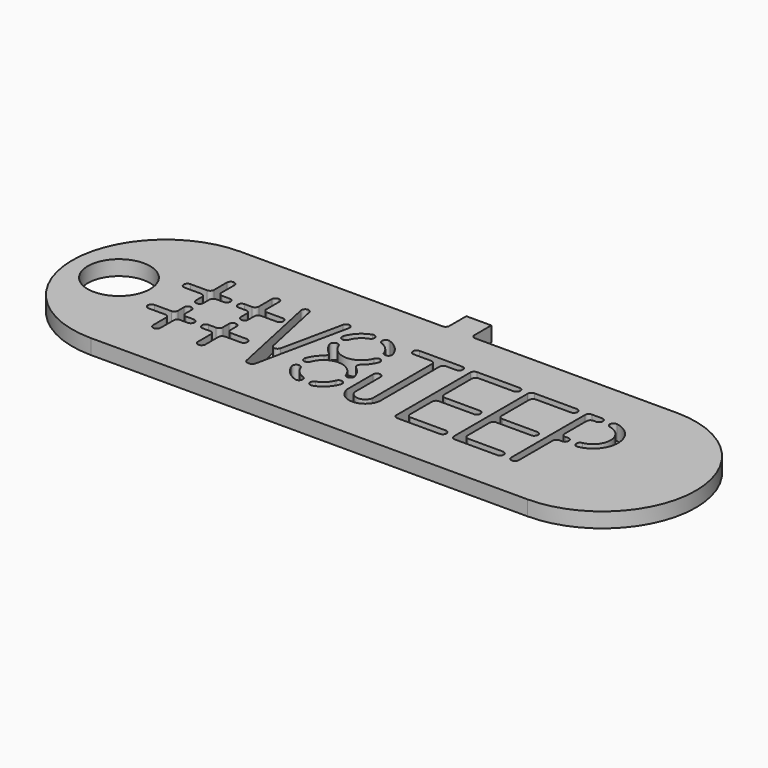
from build123d import *

# Parameters (mm, degrees)
F0_R        = 3.175
F1_DEPTH    = 1.524
F2_T1_DEPTH = 1.524
F2_T3_DEPTH = 10.4029181171
F2_T5_DEPTH = 3.429
F2_T7_DEPTH = 4.4158412882
F3_R        = 0.38
F4_R        = 0.38


# Not quite as in the source:
# - a fillet or chamfer that OpenCascade refuses, or shapes differently, is made with other operations: its cross-section is extruded or revolved along the edge and cut away or added
# - a fillet or chamfer is up to 0.001 mm smaller than in the source, because OpenCascade refuses the exact size


with BuildPart() as f1:
    # F0 (on Top) → F1 (new body)
    with BuildSketch(Plane.XY):
        with BuildLine():
            Line((30.48, 19.05), (9.525, 19.05))
            ThreePointArc((9.525, 19.05), (0, 9.525), (9.525, 0))
            Line((9.525, 0), (53.975, 0))
            ThreePointArc((53.975, 0), (63.5, 9.525), (53.975, 19.05))
            Line((53.975, 19.05), (33.02, 19.05))
            Line((33.02, 19.05), (33.02, 21.59))
            Line((33.02, 21.59), (30.48, 21.59))
            Line((30.48, 21.59), (30.48, 19.05))
        make_face()
        Polygon((9.525, 7.6261373708), (11.990133673, 7.6261373708), (11.990133673, 9.1501373708), (12.752133673, 9.1501373708), (12.752133673, 7.6261373708), (14.276133673, 7.6261373708), (14.276133673, 6.8641373708), (12.752133673, 6.8641373708), (12.752133673, 4.445), (11.990133673, 4.445), (11.990133673, 6.8641373708), (9.525, 6.8641373708), align=None, mode=Mode.SUBTRACT)
        with Locations((4.7625, 9.525)):
            Circle(F0_R, mode=Mode.SUBTRACT)
        Polygon((16.562133673, 6.8641373708), (15.038133673, 6.8641373708), (15.038133673, 7.6261373708), (16.562133673, 7.6261373708), (16.562133673, 9.1501373708), (17.324133673, 9.1501373708), (17.324133673, 7.6261373708), (19.685, 7.6261373708), (19.685, 6.8641373708), (17.324133673, 6.8641373708), (17.324133673, 4.445), (16.562133673, 4.445), align=None, mode=Mode.SUBTRACT)
        with BuildLine():
            ThreePointArc((25.6528369587, 6.6981185685), (26.1772344094, 5.7531270917), (27.1313334392, 5.245488816))
            Line((27.1313334392, 5.245488816), (27.1313334392, 4.4723545693))
            ThreePointArc((27.1313334392, 4.4723545693), (25.6382729221, 5.2144262391), (24.8776434838, 6.6981185685))
            Line((24.8776434838, 6.6981185685), (25.6528369587, 6.6981185685))
        make_face(mode=Mode.SUBTRACT)
        with BuildLine():
            Line((27.8933334392, 4.4723545693), (27.8933334392, 5.245488816))
            ThreePointArc((27.8933334392, 5.245488816), (28.8528284175, 5.7584497745), (29.3750644231, 6.7129282251))
            Line((29.3750644231, 6.7129282251), (30.1493072196, 6.7129282251))
            ThreePointArc((30.1493072196, 6.7129282251), (29.3917173839, 5.2196984943), (27.8933334392, 4.4723545693))
        make_face(mode=Mode.SUBTRACT)
        Polygon((21.6525053587, 4.445), (19.4935053587, 14.605), (20.2555053587, 14.605), (22.0335053587, 6.3180097573), (23.8115053587, 14.605), (24.5735053587, 14.605), (22.4145053587, 4.445), align=None, mode=Mode.SUBTRACT)
        with BuildLine():
            ThreePointArc((26.3764109066, 9.525), (25.3757333504, 10.3418079499), (24.876256228, 11.5330482291))
            Line((24.876256228, 11.5330482291), (25.6508718996, 11.5330482291))
            ThreePointArc((25.6508718996, 11.5330482291), (27.5215165568, 10.0330221339), (29.3776125895, 11.5510133188))
            Line((29.3776125895, 11.5510133188), (30.1511078343, 11.5510133188))
            ThreePointArc((30.1511078343, 11.5510133188), (29.6543574157, 10.3490939978), (28.6482559717, 9.525))
            ThreePointArc((28.6482559717, 9.525), (29.6615736807, 8.6911312118), (30.1545242164, 7.4749282251))
            Line((30.1545242164, 7.4749282251), (29.3824425545, 7.4749282251))
            ThreePointArc((29.3824425545, 7.4749282251), (27.5047961864, 9.0169850891), (25.6394110002, 7.4601185685))
            Line((25.6394110002, 7.4601185685), (24.8681506803, 7.4601185685))
            ThreePointArc((24.8681506803, 7.4601185685), (25.3586777482, 8.6851039905), (26.3764109066, 9.525))
        make_face(mode=Mode.SUBTRACT)
        with BuildLine():
            Line((30.9413334392, 5.8339602692), (30.9413334392, 9.525))
            Line((30.9413334392, 9.525), (31.7033334392, 9.525))
            Line((31.7033334392, 9.525), (31.7033334392, 5.8339602692))
            ThreePointArc((31.7033334392, 5.8339602692), (32.5923334392, 5.1729728532), (33.4813334392, 5.8339602692))
            Line((33.4813334392, 5.8339602692), (33.4813334392, 13.843))
            Line((33.4813334392, 13.843), (30.9413334392, 13.843))
            Line((30.9413334392, 13.843), (30.9413334392, 14.605))
            Line((30.9413334392, 14.605), (36.0213334392, 14.605))
            Line((36.0213334392, 14.605), (36.0213334392, 13.843))
            Line((36.0213334392, 13.843), (34.2433334392, 13.843))
            Line((34.2433334392, 13.843), (34.2433334392, 5.8339602692))
            ThreePointArc((34.2433334392, 5.8339602692), (32.5923334392, 4.4338967074), (30.9413334392, 5.8339602692))
        make_face(mode=Mode.SUBTRACT)
        Polygon((41.8633334392, 14.605), (41.8633334392, 13.843), (37.5453334392, 13.843), (37.5453334392, 9.5561961154), (41.8633334392, 9.5561961154), (41.8633334392, 8.7941961154), (37.5453334392, 8.7941961154), (37.5453334392, 5.207), (41.8633334392, 5.207), (41.8633334392, 4.445), (36.7833334392, 4.445), (36.7833334392, 14.605), align=None, mode=Mode.SUBTRACT)
        Polygon((42.6253334392, 4.445), (42.6253334392, 14.605), (47.7053334392, 14.605), (47.7053334392, 13.843), (43.3873334392, 13.843), (43.3873334392, 9.5561961154), (47.7053334392, 9.5561961154), (47.7053334392, 8.7941961154), (43.3873334392, 8.7941961154), (43.3873334392, 5.207), (47.7053334392, 5.207), (47.7053334392, 4.445), align=None, mode=Mode.SUBTRACT)
        Polygon((49.2293334392, 4.445), (48.4673334392, 4.445), (48.4673334392, 14.605), (50.2805225551, 14.605), (50.2805225551, 13.8435801491), (49.2293334392, 13.843), (49.2293334392, 10.287), (50.2624474466, 10.287), (50.2624474466, 9.525), (49.2293334392, 9.525), align=None, mode=Mode.SUBTRACT)
        Polygon((11.990133673, 12.1981373708), (11.990133673, 14.605), (12.752133673, 14.605), (12.752133673, 12.1981373708), (14.276133673, 12.1981373708), (14.276133673, 11.4361373708), (12.752133673, 11.4361373708), (12.752133673, 9.9121373708), (11.990133673, 9.9121373708), (11.990133673, 11.4361373708), (9.525, 11.4361373708), (9.525, 12.1981373708), align=None, mode=Mode.SUBTRACT)
        Polygon((16.562133673, 12.1981373708), (16.562133673, 14.605), (17.324133673, 14.605), (17.324133673, 12.1981373708), (19.685, 12.1981373708), (19.685, 11.4361373708), (17.324133673, 11.4361373708), (17.324133673, 9.9121373708), (16.562133673, 9.9121373708), (16.562133673, 11.4361373708), (15.038133673, 11.4361373708), (15.038133673, 12.1981373708), align=None, mode=Mode.SUBTRACT)
        with BuildLine():
            ThreePointArc((24.8693416567, 12.2950482291), (25.6185493529, 13.8158899953), (27.1330227926, 14.5778887161))
            Line((27.1330227926, 14.5778887161), (27.1330227926, 13.8048552256))
            ThreePointArc((27.1330227926, 13.8048552256), (26.1572966965, 13.2769923174), (25.6410927913, 12.2950482291))
            Line((25.6410927913, 12.2950482291), (24.8693416567, 12.2950482291))
        make_face(mode=Mode.SUBTRACT)
        with BuildLine():
            ThreePointArc((29.3800566549, 12.3130133188), (28.8621381004, 13.2822664827), (27.8950224806, 13.8041656137))
            Line((27.8950224806, 13.8041656137), (27.8950227926, 14.5774010417))
            ThreePointArc((27.8950227926, 14.5774010417), (29.4009269225, 13.8211101016), (30.1528360449, 12.3130133188))
            Line((30.1528360449, 12.3130133188), (29.3800566549, 12.3130133188))
        make_face(mode=Mode.SUBTRACT)
        with BuildLine():
            ThreePointArc((51.0073334392, 14.605), (53.5473334392, 12.065), (51.0073334392, 9.525))
            Line((51.0073334392, 9.525), (51.0073334392, 10.287))
            ThreePointArc((51.0073334392, 10.287), (52.7853334392, 12.065), (51.0073334392, 13.843))
            Line((51.0073334392, 13.843), (51.0073334392, 14.605))
        make_face(mode=Mode.SUBTRACT)
    extrude(amount=F1_DEPTH)

    # F2: fillet of radius 0.381 on 77 edges, made by hand

    # F2_s2 → F2_t1 (join)
    with BuildSketch(Plane.XY):
        with BuildLine():
            ThreePointArc((24.103035572, 14.605), (24.3991216953, 14.4637790808), (24.4757140942, 14.144805814))
            Line((24.4757140942, 14.144805814), (24.5735053587, 14.605))
            Line((24.5735053587, 14.605), (24.103035572, 14.605))
        make_face()
        with BuildLine():
            ThreePointArc((20.3201017736, 14.3039258381), (20.1870677408, 14.5203214001), (19.9475794784, 14.605))
            Line((19.9475794784, 14.605), (20.2555053587, 14.605))
            Line((20.2555053587, 14.605), (20.3201017736, 14.3039258381))
        make_face()
        with BuildLine():
            ThreePointArc((23.7469089438, 14.3039258381), (23.8799429766, 14.5203214001), (24.119431239, 14.605))
            Line((24.119431239, 14.605), (23.8115053587, 14.605))
            Line((23.8115053587, 14.605), (23.7469089438, 14.3039258381))
        make_face()
        with BuildLine():
            ThreePointArc((19.5912966232, 14.144805814), (19.6678890221, 14.4637790808), (19.9639751454, 14.605))
            Line((19.9639751454, 14.605), (19.4935053587, 14.605))
            Line((19.4935053587, 14.605), (19.5912966232, 14.144805814))
        make_face()
        with BuildLine():
            ThreePointArc((21.9610501454, 4.445), (21.7212710646, 4.5299138767), (21.5883716232, 4.746805814))
            Line((21.5883716232, 4.746805814), (21.6525053587, 4.445))
            Line((21.6525053587, 4.445), (21.9610501454, 4.445))
        make_face()
        with BuildLine():
            ThreePointArc((22.4786390942, 4.746805814), (22.3457396527, 4.5299138767), (22.105960572, 4.445))
            Line((22.105960572, 4.445), (22.4145053587, 4.445))
            Line((22.4145053587, 4.445), (22.4786390942, 4.746805814))
        make_face()
        with BuildLine():
            ThreePointArc((35.6403334392, 14.605), (35.9097411228, 14.4934076836), (36.0213334392, 14.224))
            Line((36.0213334392, 14.224), (36.0213334392, 14.605))
            Line((36.0213334392, 14.605), (35.6403334392, 14.605))
        make_face()
        with BuildLine():
            ThreePointArc((36.0213334392, 14.224), (35.9097411228, 13.9545923164), (35.6403334392, 13.843))
            Line((35.6403334392, 13.843), (36.0213334392, 13.843))
            Line((36.0213334392, 13.843), (36.0213334392, 14.224))
        make_face()
        with BuildLine():
            ThreePointArc((31.3223334392, 13.843), (31.0529257555, 13.9545923164), (30.9413334392, 14.224))
            Line((30.9413334392, 14.224), (30.9413334392, 13.843))
            Line((30.9413334392, 13.843), (31.3223334392, 13.843))
        make_face()
        with BuildLine():
            ThreePointArc((30.9413334392, 14.224), (31.0529257555, 14.4934076836), (31.3223334392, 14.605))
            Line((31.3223334392, 14.605), (30.9413334392, 14.605))
            Line((30.9413334392, 14.605), (30.9413334392, 14.224))
        make_face()
        with BuildLine():
            ThreePointArc((30.9413334392, 9.144), (31.0529257555, 9.4134076836), (31.3223334392, 9.525))
            Line((31.3223334392, 9.525), (30.9413334392, 9.525))
            Line((30.9413334392, 9.525), (30.9413334392, 9.144))
        make_face()
        with BuildLine():
            ThreePointArc((31.3223334392, 9.525), (31.5917411228, 9.4134076836), (31.7033334392, 9.144))
            Line((31.7033334392, 9.144), (31.7033334392, 9.525))
            Line((31.7033334392, 9.525), (31.3223334392, 9.525))
        make_face()
        with BuildLine():
            ThreePointArc((41.4823334392, 14.605), (41.7517411228, 14.4934076836), (41.8633334392, 14.224))
            Line((41.8633334392, 14.224), (41.8633334392, 14.605))
            Line((41.8633334392, 14.605), (41.4823334392, 14.605))
        make_face()
        with BuildLine():
            ThreePointArc((41.4823334392, 9.5561961154), (41.7517411228, 9.444603799), (41.8633334392, 9.1751961154))
            Line((41.8633334392, 9.1751961154), (41.8633334392, 9.5561961154))
            Line((41.8633334392, 9.5561961154), (41.4823334392, 9.5561961154))
        make_face()
        with BuildLine():
            ThreePointArc((41.4823334392, 5.207), (41.7517411228, 5.0954076836), (41.8633334392, 4.826))
            Line((41.8633334392, 4.826), (41.8633334392, 5.207))
            Line((41.8633334392, 5.207), (41.4823334392, 5.207))
        make_face()
        with BuildLine():
            ThreePointArc((37.1643334392, 14.605), (36.8949257555, 14.4934076836), (36.7833334392, 14.224))
            Line((36.7833334392, 14.224), (36.7833334392, 14.605))
            Line((36.7833334392, 14.605), (37.1643334392, 14.605))
        make_face()
        with BuildLine():
            ThreePointArc((37.1643334392, 4.445), (36.8949257555, 4.5565923164), (36.7833334392, 4.826))
            Line((36.7833334392, 4.826), (36.7833334392, 4.445))
            Line((36.7833334392, 4.445), (37.1643334392, 4.445))
        make_face()
        with BuildLine():
            ThreePointArc((42.6253334392, 4.826), (42.7369257555, 4.5565923164), (43.0063334392, 4.445))
            Line((43.0063334392, 4.445), (42.6253334392, 4.445))
            Line((42.6253334392, 4.445), (42.6253334392, 4.826))
        make_face()
        with BuildLine():
            ThreePointArc((41.8633334392, 4.826), (41.7517411228, 4.5565923164), (41.4823334392, 4.445))
            Line((41.4823334392, 4.445), (41.8633334392, 4.445))
            Line((41.8633334392, 4.445), (41.8633334392, 4.826))
        make_face()
        with BuildLine():
            ThreePointArc((41.8633334392, 9.1751961154), (41.7517411228, 8.9057884318), (41.4823334392, 8.7941961154))
            Line((41.4823334392, 8.7941961154), (41.8633334392, 8.7941961154))
            Line((41.8633334392, 8.7941961154), (41.8633334392, 9.1751961154))
        make_face()
        with BuildLine():
            ThreePointArc((41.8633334392, 14.224), (41.7517411228, 13.9545923164), (41.4823334392, 13.843))
            Line((41.4823334392, 13.843), (41.8633334392, 13.843))
            Line((41.8633334392, 13.843), (41.8633334392, 14.224))
        make_face()
        with BuildLine():
            ThreePointArc((47.7053334392, 4.826), (47.5937411228, 4.5565923164), (47.3243334392, 4.445))
            Line((47.3243334392, 4.445), (47.7053334392, 4.445))
            Line((47.7053334392, 4.445), (47.7053334392, 4.826))
        make_face()
        with BuildLine():
            ThreePointArc((47.7053334392, 9.1751961154), (47.5937411228, 8.9057884318), (47.3243334392, 8.7941961154))
            Line((47.3243334392, 8.7941961154), (47.7053334392, 8.7941961154))
            Line((47.7053334392, 8.7941961154), (47.7053334392, 9.1751961154))
        make_face()
        with BuildLine():
            ThreePointArc((47.7053334392, 14.224), (47.5937411228, 13.9545923164), (47.3243334392, 13.843))
            Line((47.3243334392, 13.843), (47.7053334392, 13.843))
            Line((47.7053334392, 13.843), (47.7053334392, 14.224))
        make_face()
        with BuildLine():
            ThreePointArc((42.6253334392, 14.224), (42.7369257555, 14.4934076836), (43.0063334392, 14.605))
            Line((43.0063334392, 14.605), (42.6253334392, 14.605))
            Line((42.6253334392, 14.605), (42.6253334392, 14.224))
        make_face()
        with BuildLine():
            ThreePointArc((47.3243334392, 5.207), (47.5937411228, 5.0954076836), (47.7053334392, 4.826))
            Line((47.7053334392, 4.826), (47.7053334392, 5.207))
            Line((47.7053334392, 5.207), (47.3243334392, 5.207))
        make_face()
        with BuildLine():
            ThreePointArc((47.3243334392, 9.5561961154), (47.5937411228, 9.444603799), (47.7053334392, 9.1751961154))
            Line((47.7053334392, 9.1751961154), (47.7053334392, 9.5561961154))
            Line((47.7053334392, 9.5561961154), (47.3243334392, 9.5561961154))
        make_face()
        with BuildLine():
            ThreePointArc((47.3243334392, 14.605), (47.5937411228, 14.4934076836), (47.7053334392, 14.224))
            Line((47.7053334392, 14.224), (47.7053334392, 14.605))
            Line((47.7053334392, 14.605), (47.3243334392, 14.605))
        make_face()
        with BuildLine():
            ThreePointArc((49.8995225551, 14.605), (50.1689302387, 14.4934076836), (50.2805225551, 14.224))
            Line((50.2805225551, 14.224), (50.2805225551, 14.605))
            Line((50.2805225551, 14.605), (49.8995225551, 14.605))
        make_face()
        with BuildLine():
            ThreePointArc((49.8814474466, 10.287), (50.1508551302, 10.1754076836), (50.2624474466, 9.906))
            Line((50.2624474466, 9.906), (50.2624474466, 10.287))
            Line((50.2624474466, 10.287), (49.8814474466, 10.287))
        make_face()
        with BuildLine():
            ThreePointArc((50.2624474466, 9.906), (50.1508551302, 9.6365923164), (49.8814474466, 9.525))
            Line((49.8814474466, 9.525), (50.2624474466, 9.525))
            Line((50.2624474466, 9.525), (50.2624474466, 9.906))
        make_face()
        with BuildLine():
            ThreePointArc((48.8483334392, 4.445), (49.1177411228, 4.5565923164), (49.2293334392, 4.826))
            Line((49.2293334392, 4.826), (49.2293334392, 4.445))
            Line((49.2293334392, 4.445), (48.8483334392, 4.445))
        make_face()
        with BuildLine():
            ThreePointArc((51.4555687333, 9.5648629795), (51.14384995, 9.6476698719), (51.0073334392, 9.9398835326))
            Line((51.0073334392, 9.9398835326), (51.0073334392, 9.525))
            ThreePointArc((51.0073334392, 9.525), (51.2323356258, 9.5349853724), (51.4555687333, 9.5648629795))
        make_face()
        with BuildLine():
            ThreePointArc((51.321098145, 13.8150959143), (51.0961197784, 13.9456329782), (51.0073334392, 14.1901164674))
            Line((51.0073334392, 14.1901164674), (51.0073334392, 13.843))
            ThreePointArc((51.0073334392, 13.843), (51.1648349698, 13.8360102393), (51.321098145, 13.8150959143))
        make_face()
        with BuildLine():
            ThreePointArc((51.321098145, 10.3149040857), (51.0961197784, 10.1843670218), (51.0073334392, 9.9398835326))
            Line((51.0073334392, 9.9398835326), (51.0073334392, 10.287))
            ThreePointArc((51.0073334392, 10.287), (51.1648349698, 10.2939897607), (51.321098145, 10.3149040857))
        make_face()
        with BuildLine():
            ThreePointArc((51.0073334392, 14.1901164674), (51.14384995, 14.4823301281), (51.4555687333, 14.5651370205))
            ThreePointArc((51.4555687333, 14.5651370205), (51.2323356258, 14.5950146276), (51.0073334392, 14.605))
            Line((51.0073334392, 14.605), (51.0073334392, 14.1901164674))
        make_face()
        with BuildLine():
            ThreePointArc((48.4673334392, 14.224), (48.5789257555, 14.4934076836), (48.8483334392, 14.605))
            Line((48.8483334392, 14.605), (48.4673334392, 14.605))
            Line((48.4673334392, 14.605), (48.4673334392, 14.224))
        make_face()
        with BuildLine():
            ThreePointArc((48.8483334392, 4.445), (48.5789257555, 4.5565923164), (48.4673334392, 4.826))
            Line((48.4673334392, 4.826), (48.4673334392, 4.445))
            Line((48.4673334392, 4.445), (48.8483334392, 4.445))
        make_face()
        with BuildLine():
            ThreePointArc((29.6738992595, 7.4749282251), (29.4526284326, 7.5457666202), (29.3136382895, 7.7319401876))
            ThreePointArc((29.3136382895, 7.7319401876), (29.3525328615, 7.6046368702), (29.3824425545, 7.4749282251))
            Line((29.3824425545, 7.4749282251), (29.6738992595, 7.4749282251))
        make_face()
        with BuildLine():
            ThreePointArc((30.0341602296, 7.9799162626), (29.9840608644, 7.6346573982), (29.6738992595, 7.4749282251))
            Line((29.6738992595, 7.4749282251), (30.1545242164, 7.4749282251))
            ThreePointArc((30.1545242164, 7.4749282251), (30.1066585131, 7.7303578338), (30.0341602296, 7.9799162626))
        make_face()
        with BuildLine():
            ThreePointArc((29.6611200796, 6.7129282251), (29.9731261354, 6.5505905702), (30.0192511863, 6.2019162626))
            ThreePointArc((30.0192511863, 6.2019162626), (30.0969394668, 6.4542001203), (30.1493072196, 6.7129282251))
            Line((30.1493072196, 6.7129282251), (29.6611200796, 6.7129282251))
        make_face()
        with BuildLine():
            ThreePointArc((27.8933334392, 4.9567385309), (28.0543629866, 4.6456533336), (28.4013334392, 4.5975282861))
            ThreePointArc((28.4013334392, 4.5975282861), (28.150410327, 4.5224543091), (27.8933334392, 4.4723545693))
            Line((27.8933334392, 4.4723545693), (27.8933334392, 4.9567385309))
        make_face()
        with BuildLine():
            ThreePointArc((27.8933334392, 4.9567385309), (27.9632482418, 5.1767089835), (28.1473334392, 5.3159487758))
            ThreePointArc((28.1473334392, 5.3159487758), (28.0215535796, 5.2763203306), (27.8933334392, 5.245488816))
            Line((27.8933334392, 5.245488816), (27.8933334392, 4.9567385309))
        make_face()
        with BuildLine():
            ThreePointArc((29.3029889728, 6.4619401876), (29.4424577345, 6.6439342809), (29.6611200796, 6.7129282251))
            Line((29.6611200796, 6.7129282251), (29.3750644231, 6.7129282251))
            ThreePointArc((29.3750644231, 6.7129282251), (29.3433323497, 6.5861977658), (29.3029889728, 6.4619401876))
        make_face()
        with BuildLine():
            ThreePointArc((25.3689810393, 6.6981185685), (25.5865655391, 6.6298772382), (25.7262064393, 6.4495988071))
            ThreePointArc((25.7262064393, 6.4495988071), (25.6852912508, 6.5726097498), (25.6528369587, 6.6981185685))
            Line((25.6528369587, 6.6981185685), (25.3689810393, 6.6981185685))
        make_face()
        with BuildLine():
            ThreePointArc((27.1313334392, 4.9567385309), (27.0614186365, 5.1767089835), (26.8773334392, 5.3159487758))
            ThreePointArc((26.8773334392, 5.3159487758), (27.0031132987, 5.2763203306), (27.1313334392, 5.245488816))
            Line((27.1313334392, 5.245488816), (27.1313334392, 4.9567385309))
        make_face()
        with BuildLine():
            ThreePointArc((27.1313334392, 4.9567385309), (26.9703038917, 4.6456533336), (26.6233334392, 4.5975282861))
            ThreePointArc((26.6233334392, 4.5975282861), (26.8742565513, 4.5224543091), (27.1313334392, 4.4723545693))
            Line((27.1313334392, 4.4723545693), (27.1313334392, 4.9567385309))
        make_face()
        with BuildLine():
            ThreePointArc((25.0117556393, 6.1846383299), (25.0562223697, 6.5347030683), (25.3689810393, 6.6981185685))
            Line((25.3689810393, 6.6981185685), (24.8776434838, 6.6981185685))
            ThreePointArc((24.8776434838, 6.6981185685), (24.9318956433, 6.4380342873), (25.0117556393, 6.1846383299))
        make_face()
        with BuildLine():
            ThreePointArc((25.3457273114, 7.4601185685), (25.5680581132, 7.5317158947), (25.7068283327, 7.7195988071))
            ThreePointArc((25.7068283327, 7.7195988071), (25.6685493411, 7.5910461353), (25.6394110002, 7.4601185685))
            Line((25.6394110002, 7.4601185685), (25.3457273114, 7.4601185685))
        make_face()
        with BuildLine():
            ThreePointArc((25.3457273114, 7.4601185685), (25.0363246376, 7.6187877667), (24.9846262901, 7.9626383299))
            ThreePointArc((24.9846262901, 7.9626383299), (24.9142104951, 7.7142011021), (24.8681506803, 7.4601185685))
            Line((24.8681506803, 7.4601185685), (25.3457273114, 7.4601185685))
        make_face()
        with BuildLine():
            ThreePointArc((25.0079167025, 11.0210562673), (25.0533854328, 11.3702832659), (25.365690522, 11.5330482291))
            Line((25.365690522, 11.5330482291), (24.876256228, 11.5330482291))
            ThreePointArc((24.876256228, 11.5330482291), (24.9293693571, 11.2737820006), (25.0079167025, 11.0210562673))
        make_face()
        with BuildLine():
            ThreePointArc((25.365690522, 11.5330482291), (25.5839255588, 11.4643533183), (25.7234643415, 11.2830401909))
            ThreePointArc((25.7234643415, 11.2830401909), (25.6828924193, 11.4068027155), (25.6508718996, 11.5330482291))
            Line((25.6508718996, 11.5330482291), (25.365690522, 11.5330482291))
        make_face()
        with BuildLine():
            ThreePointArc((29.3066130179, 11.298011099), (29.4459309577, 11.4814038728), (29.6654689336, 11.5510133188))
            Line((29.6654689336, 11.5510133188), (29.3776125895, 11.5510133188))
            ThreePointArc((29.3776125895, 11.5510133188), (29.3464803944, 11.4232865395), (29.3066130179, 11.298011099))
        make_face()
        with BuildLine():
            ThreePointArc((29.6654689336, 11.5510133188), (29.9768594876, 11.3895512947), (30.0243248494, 11.0420155386))
            ThreePointArc((30.0243248494, 11.0420155386), (30.1002605596, 11.2933898701), (30.1511078343, 11.5510133188))
            Line((30.1511078343, 11.5510133188), (29.6654689336, 11.5510133188))
        make_face()
        with BuildLine():
            ThreePointArc((26.6253043515, 14.4531676679), (26.97211513, 14.404856977), (27.1330227926, 14.0938580011))
            Line((27.1330227926, 14.0938580011), (27.1330227926, 14.5778887161))
            ThreePointArc((27.1330227926, 14.5778887161), (26.8761000578, 14.5279992441), (26.6253043515, 14.4531676679))
        make_face()
        with BuildLine():
            ThreePointArc((26.8787412337, 13.7345483342), (27.0630217685, 13.8737656637), (27.1330227926, 14.0938580011))
            Line((27.1330227926, 14.0938580011), (27.1330227926, 13.8048552256))
            ThreePointArc((27.1330227926, 13.8048552256), (27.0046634561, 13.7741089805), (26.8787412337, 13.7345483342))
        make_face()
        with BuildLine():
            ThreePointArc((25.7093496446, 12.5530401909), (25.5704451695, 12.3661877262), (25.3487528856, 12.2950482291))
            Line((25.3487528856, 12.2950482291), (25.6410927913, 12.2950482291))
            ThreePointArc((25.6410927913, 12.2950482291), (25.6706979496, 12.4252409297), (25.7093496446, 12.5530401909))
        make_face()
        with BuildLine():
            ThreePointArc((25.3487528856, 12.2950482291), (25.0388923827, 12.4543559452), (24.9881561267, 12.7990562673))
            ThreePointArc((24.9881561267, 12.7990562673), (24.9164876927, 12.5499426939), (24.8693416567, 12.2950482291))
            Line((24.8693416567, 12.2950482291), (25.3487528856, 12.2950482291))
        make_face()
        with BuildLine():
            ThreePointArc((28.1487410707, 13.7335529306), (27.9648511678, 13.8728150652), (27.895022597, 14.0926636705))
            Line((27.895022597, 14.0926636705), (27.8950224806, 13.8041656137))
            ThreePointArc((27.8950224806, 13.8041656137), (28.0231034901, 13.7732490172), (28.1487410707, 13.7335529306))
        make_face()
        with BuildLine():
            ThreePointArc((29.3101407189, 12.568011099), (29.4493000943, 12.3832337782), (29.6697021749, 12.3130133188))
            Line((29.6697021749, 12.3130133188), (29.3800566549, 12.3130133188))
            ThreePointArc((29.3800566549, 12.3130133188), (29.349528154, 12.4417266914), (29.3101407189, 12.568011099))
        make_face()
        with BuildLine():
            ThreePointArc((27.895022597, 14.0926636705), (28.0561741455, 14.4038349459), (28.4033041233, 14.4517741028))
            ThreePointArc((28.4033041233, 14.4517741028), (28.1522537504, 14.5270907661), (27.8950227926, 14.5774010417))
            Line((27.8950227926, 14.5774010417), (27.895022597, 14.0926636705))
        make_face()
        with BuildLine():
            ThreePointArc((30.0292636308, 12.8200155386), (29.9804817155, 12.4736112382), (29.6697021749, 12.3130133188))
            Line((29.6697021749, 12.3130133188), (30.1528360449, 12.3130133188))
            ThreePointArc((30.1528360449, 12.3130133188), (30.1034801115, 12.569544078), (30.0292636308, 12.8200155386))
        make_face()
        with BuildLine():
            ThreePointArc((30.099, 19.05), (30.3684076836, 19.1615923164), (30.48, 19.431))
            Line((30.48, 19.431), (30.48, 19.05))
            Line((30.48, 19.05), (30.099, 19.05))
        make_face()
        with BuildLine():
            ThreePointArc((33.401, 19.05), (33.1315923164, 19.1615923164), (33.02, 19.431))
            Line((33.02, 19.431), (33.02, 19.05))
            Line((33.02, 19.05), (33.401, 19.05))
        make_face()
    extrude(amount=F2_T1_DEPTH)

    # F2_s4 → F2_t3 (cut)
    with BuildSketch(Plane.XY.offset(-4.4394590586)):
        with BuildLine():
            ThreePointArc((22.4060276539, 8.0542800752), (22.0335053587, 7.7532059134), (21.6609830635, 8.0542800752))
            Line((21.6609830635, 8.0542800752), (22.0335053587, 6.3180097573))
            Line((22.0335053587, 6.3180097573), (22.4060276539, 8.0542800752))
        make_face()
    extrude(amount=F2_T3_DEPTH, mode=Mode.SUBTRACT)

    # F2_s6 → F2_t5 (cut)
    with BuildSketch(Plane.XY.offset(-0.9525)):
        with BuildLine():
            ThreePointArc((33.1003334392, 13.843), (33.3697411228, 13.7314076836), (33.4813334392, 13.462))
            Line((33.4813334392, 13.462), (33.4813334392, 13.843))
            Line((33.4813334392, 13.843), (33.1003334392, 13.843))
        make_face()
        with BuildLine():
            ThreePointArc((34.2433334392, 13.462), (34.3549257555, 13.7314076836), (34.6243334392, 13.843))
            Line((34.6243334392, 13.843), (34.2433334392, 13.843))
            Line((34.2433334392, 13.843), (34.2433334392, 13.462))
        make_face()
        with BuildLine():
            ThreePointArc((37.9263334392, 5.207), (37.6569257555, 5.3185923164), (37.5453334392, 5.588))
            Line((37.5453334392, 5.588), (37.5453334392, 5.207))
            Line((37.5453334392, 5.207), (37.9263334392, 5.207))
        make_face()
        with BuildLine():
            ThreePointArc((37.9263334392, 9.5561961154), (37.6569257555, 9.6677884318), (37.5453334392, 9.9371961154))
            Line((37.5453334392, 9.9371961154), (37.5453334392, 9.5561961154))
            Line((37.5453334392, 9.5561961154), (37.9263334392, 9.5561961154))
        make_face()
        with BuildLine():
            ThreePointArc((37.5453334392, 8.4131961154), (37.6569257555, 8.682603799), (37.9263334392, 8.7941961154))
            Line((37.9263334392, 8.7941961154), (37.5453334392, 8.7941961154))
            Line((37.5453334392, 8.7941961154), (37.5453334392, 8.4131961154))
        make_face()
        with BuildLine():
            ThreePointArc((37.5453334392, 13.462), (37.6569257555, 13.7314076836), (37.9263334392, 13.843))
            Line((37.9263334392, 13.843), (37.5453334392, 13.843))
            Line((37.5453334392, 13.843), (37.5453334392, 13.462))
        make_face()
        with BuildLine():
            ThreePointArc((43.3873334392, 13.462), (43.4989257555, 13.7314076836), (43.7683334392, 13.843))
            Line((43.7683334392, 13.843), (43.3873334392, 13.843))
            Line((43.3873334392, 13.843), (43.3873334392, 13.462))
        make_face()
        with BuildLine():
            ThreePointArc((43.7683334392, 9.5561961154), (43.4989257555, 9.6677884318), (43.3873334392, 9.9371961154))
            Line((43.3873334392, 9.9371961154), (43.3873334392, 9.5561961154))
            Line((43.3873334392, 9.5561961154), (43.7683334392, 9.5561961154))
        make_face()
        with BuildLine():
            ThreePointArc((43.3873334392, 8.4131961154), (43.4989257555, 8.682603799), (43.7683334392, 8.7941961154))
            Line((43.7683334392, 8.7941961154), (43.3873334392, 8.7941961154))
            Line((43.3873334392, 8.7941961154), (43.3873334392, 8.4131961154))
        make_face()
        with BuildLine():
            ThreePointArc((43.7683334392, 5.207), (43.4989257555, 5.3185923164), (43.3873334392, 5.588))
            Line((43.3873334392, 5.588), (43.3873334392, 5.207))
            Line((43.3873334392, 5.207), (43.7683334392, 5.207))
        make_face()
    extrude(amount=F2_T5_DEPTH, mode=Mode.SUBTRACT)

    # F2_s8 → F2_t7 (cut)
    with BuildSketch(Plane.XY.offset(-1.4459206441)):
        with BuildLine():
            ThreePointArc((25.8829210882, 9.826625), (26.0311478952, 9.525), (25.8829210882, 9.223375))
            ThreePointArc((25.8829210882, 9.223375), (26.1214654855, 9.387604389), (26.3764109066, 9.525))
            ThreePointArc((26.3764109066, 9.525), (26.1214654855, 9.662395611), (25.8829210882, 9.826625))
        make_face()
        with BuildLine():
            ThreePointArc((29.1417457901, 9.223375), (28.9935189831, 9.525), (29.1417457901, 9.826625))
            ThreePointArc((29.1417457901, 9.826625), (28.9032013929, 9.662395611), (28.6482559717, 9.525))
            ThreePointArc((28.6482559717, 9.525), (28.9032013929, 9.387604389), (29.1417457901, 9.223375))
        make_face()
    extrude(amount=F2_T7_DEPTH, mode=Mode.SUBTRACT)

    # F3 (radius 0.381 in the source; OpenCascade refuses exactly that, so slightly less here)
    f3_edges = [f1.edges().sort_by_distance(p)[0] for p in [
        (19.685, 11.436137, 0.762),
        (19.685, 6.864137, 0.762),
        (17.324134, 4.445, 0.762),
        (17.324134, 12.198137, 0.762),
        (17.324134, 11.436137, 0.762),
        (17.324134, 7.626137, 0.762),
        (17.324134, 6.864137, 0.762),
        (16.562134, 6.864137, 0.762),
        (16.562134, 11.436137, 0.762),
        (12.752134, 11.436137, 0.762),
        (12.752134, 12.198137, 0.762),
        (11.990134, 11.436137, 0.762),
        (14.276134, 11.436137, 0.762),
        (12.752134, 9.912137, 0.762),
        (14.276134, 6.864137, 0.762),
        (12.752134, 7.626137, 0.762),
        (12.752134, 6.864137, 0.762),
        (11.990134, 6.864137, 0.762),
        (12.752134, 4.445, 0.762),
        (16.562134, 12.198137, 0.762),
        (15.038134, 12.198137, 0.762),
        (16.562134, 14.605, 0.762),
        (16.562134, 9.150137, 0.762),
        (16.562134, 7.626137, 0.762),
        (15.038134, 7.626137, 0.762),
        (11.990134, 12.198137, 0.762),
        (9.525, 12.198137, 0.762),
        (11.990134, 14.605, 0.762),
        (11.990134, 9.150137, 0.762),
        (11.990134, 7.626137, 0.762),
        (9.525, 7.626137, 0.762),
        (9.525, 6.864137, 0.762),
        (15.038134, 6.864137, 0.762),
        (11.990134, 4.445, 0.762),
        (9.525, 11.436137, 0.762),
        (12.752134, 14.605, 0.762),
        (19.685, 7.626137, 0.762),
        (19.685, 12.198137, 0.762),
        (17.324134, 14.605, 0.762),
        (14.276134, 7.626137, 0.762),
        (14.276134, 12.198137, 0.762),
        (11.990134, 9.912137, 0.762),
        (12.752134, 9.150137, 0.762),
        (15.038134, 11.436137, 0.762),
        (16.562134, 9.912137, 0.762),
        (17.324134, 9.150137, 0.762),
        (17.324134, 9.912137, 0.762),
        (16.562134, 4.445, 0.762),
    ]]
    fillet(f3_edges, radius=F3_R)

    # F4 (radius 0.381 in the source; OpenCascade refuses exactly that, so slightly less here)
    f4_edges = [f1.edges().sort_by_distance(p)[0] for p in [
        (50.280523, 13.84358, 0.762),
        (49.229333, 13.843, 0.762),
        (49.229333, 10.287, 0.762),
        (49.229333, 9.525, 0.762),
    ]]
    fillet(f4_edges, radius=F4_R)


solid = f1.part
